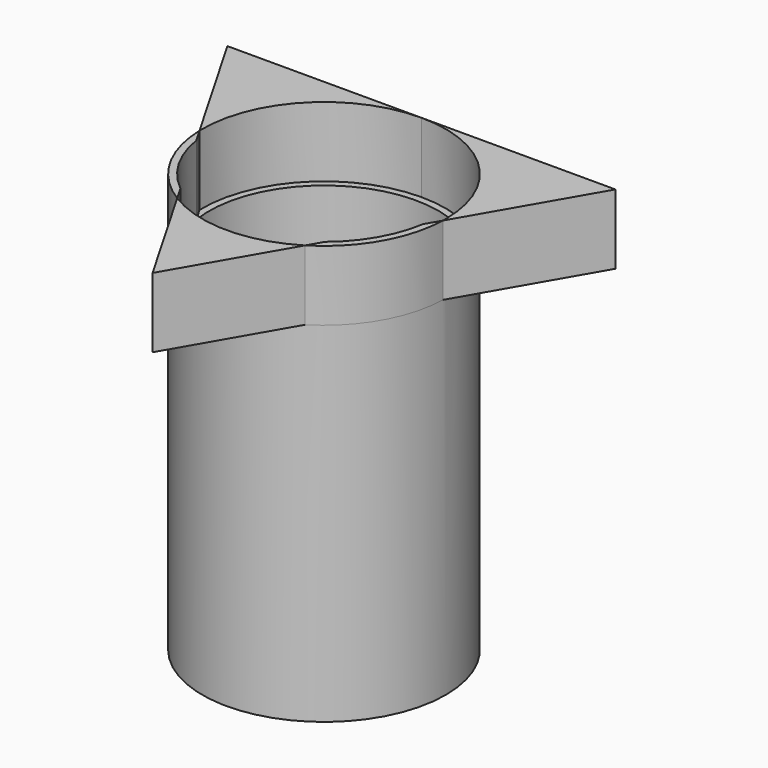
from build123d import *

# Parameters (mm, degrees)
F0_R     = 44.2783110884
F1_DEPTH = 127
F2_T     = -2.54
F4_DEPTH = 25.4
F5_DEPTH = 25.4


# Not quite as in the source:
# - after a boolean that leaves OpenCascade's solid faulty, fix() repairs it


with BuildPart() as f1:
    # F0 (on Top) → F1 (new body)
    with BuildSketch(Plane.XY):
        Circle(F0_R)
    extrude(amount=F1_DEPTH)

    # F2
    f2_openings = [f1.faces().sort_by_distance(p)[0] for p in [
        (0, 0, 127),
    ]]
    offset(amount=F2_T, openings=f2_openings)

    # F3 (on face) → F4, piece 4 (join)
    with BuildSketch(Plane.XY.offset(127)):
        with BuildLine():
            Line((-41.2220744903, -6.5442484079), (-44.2597224544, -1.2828877987))
            ThreePointArc((-44.2597224543, -1.2828877987), (-38.3461422392, -22.1391555442), (-23.2408746511, -37.6886001106))
            Line((-23.2408746511, -37.6886001106), (-26.2785226151, -32.4272395014))
            ThreePointArc((-26.2785226151, -32.4272395014), (-36.1464377136, -20.8691555442), (-41.2220744903, -6.5442484079))
        make_face()
        with BuildLine():
            ThreePointArc((23.2408746511, -37.6886001106), (38.3461422392, -22.1391555442), (44.2597224543, -1.2828877987))
            Line((44.2597224544, -1.2828877987), (41.2220744903, -6.5442484079))
            ThreePointArc((41.2220744903, -6.5442484079), (36.1464377136, -20.8691555442), (26.2785226151, -32.4272395014))
            Line((26.2785226151, -32.4272395014), (23.2408746511, -37.6886001106))
        make_face()
    extrude(amount=F4_DEPTH)

    add(f1.part.fix(), mode=Mode.REPLACE)


with BuildPart() as f4:
    # F3 (on face) → F4 (new body)
    with BuildSketch(Plane.XY.offset(127)):
        with BuildLine():
            Line((-1.56e-08, 44.2783110884), (-70.5644928964, 44.2783110884))
            Line((-70.5644928964, 44.2783110884), (-44.2597224544, -1.2828877987))
            ThreePointArc((-44.2597224543, -1.2828877987), (-31.7598247679, 30.8525908726), (-1.56e-08, 44.2783110884))
        make_face()
    extrude(amount=F4_DEPTH)


with BuildPart() as f4b:
    # F3 (on face) → F4, piece 2 (new body)
    with BuildSketch(Plane.XY.offset(127)):
        with BuildLine():
            Line((70.5644928964, 44.2783110884), (-1.56e-08, 44.2783110884))
            ThreePointArc((-1.56e-08, 44.2783110884), (31.3094940246, 31.3094940356), (44.2783110884, 0))
            ThreePointArc((44.2783110884, 0), (44.273663686, -0.6415112317), (44.2597224543, -1.2828877987))
            Line((44.2597224544, -1.2828877987), (70.5644928964, 44.2783110884))
        make_face()
    extrude(amount=F4_DEPTH)


with BuildPart() as f4c:
    # F3 (on face) → F4, piece 3 (new body)
    with BuildSketch(Plane.XY.offset(127)):
        with BuildLine():
            ThreePointArc((23.2408746511, -37.6886001106), (0, -44.2783110884), (-23.2408746511, -37.6886001106))
            Line((-23.2408746511, -37.6886001106), (0, -77.9429758185))
            Line((0, -77.9429758185), (23.2408746511, -37.6886001106))
        make_face()
    extrude(amount=F4_DEPTH)


with BuildPart() as f5:
    # F3 (on face) → F5 (new body)
    with BuildSketch(Plane.XY.offset(127)):
        with BuildLine():
            Line((70.5644928964, 44.2783110884), (-1.56e-08, 44.2783110884))
            ThreePointArc((-1.56e-08, 44.2783110884), (31.3094940246, 31.3094940356), (44.2783110884, 0))
            ThreePointArc((44.2783110884, 0), (44.273663686, -0.6415112317), (44.2597224543, -1.2828877987))
            Line((44.2597224544, -1.2828877987), (70.5644928964, 44.2783110884))
        make_face()
    extrude(amount=F5_DEPTH)


with BuildPart() as f5b:
    # F3 (on face) → F5, piece 2 (new body)
    with BuildSketch(Plane.XY.offset(127)):
        with BuildLine():
            Line((-1.56e-08, 44.2783110884), (-70.5644928964, 44.2783110884))
            Line((-70.5644928964, 44.2783110884), (-44.2597224544, -1.2828877987))
            ThreePointArc((-44.2597224543, -1.2828877987), (-31.7598247679, 30.8525908726), (-1.56e-08, 44.2783110884))
        make_face()
    extrude(amount=F5_DEPTH)


with BuildPart() as f5c:
    # F3 (on face) → F5, piece 3 (new body)
    with BuildSketch(Plane.XY.offset(127)):
        with BuildLine():
            ThreePointArc((23.2408746511, -37.6886001106), (0, -44.2783110884), (-23.2408746511, -37.6886001106))
            Line((-23.2408746511, -37.6886001106), (0, -77.9429758185))
            Line((0, -77.9429758185), (23.2408746511, -37.6886001106))
        make_face()
    extrude(amount=F5_DEPTH)


solid = Compound([f1.part, f4.part, f4b.part, f4c.part, f5.part, f5b.part, f5c.part])
